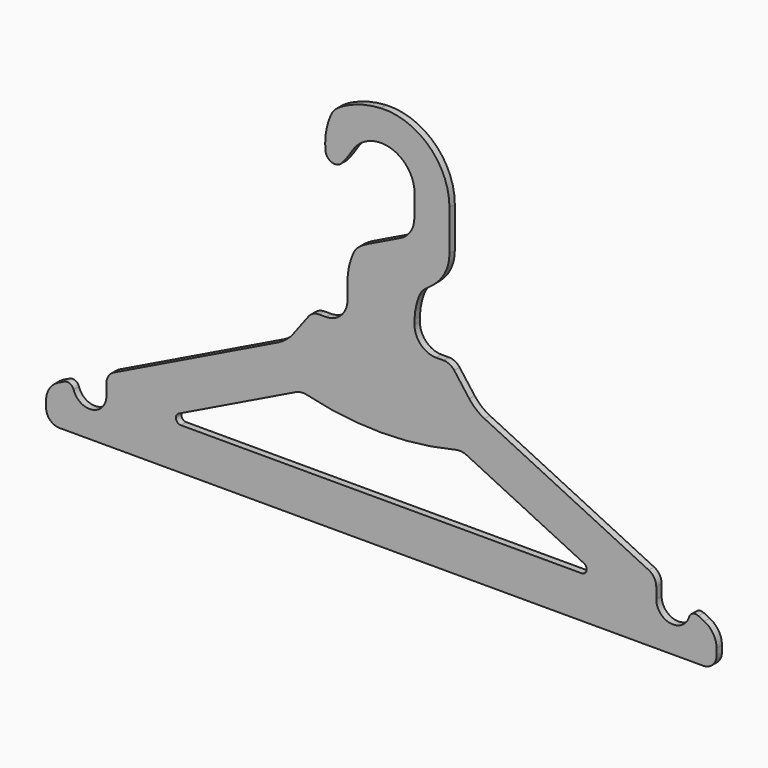
from build123d import *

# Parameters (mm, degrees)
F4_DEPTH = 4
F5_DEPTH = 25
F6_DEPTH = 4


# Not quite as in the source:
# - ends of sketch curves that miss each other by under 0.0002 mm in the source are joined


with BuildPart() as f4:
    # F1 (on Front) → F4 (new body)
    with BuildSketch(Plane.XZ):
        with BuildLine():
            Line((-192, 0), (0, 0))
            Line((0, 0), (192, 0))
            ThreePointArc((192, 0), (197.656854, 2.343146), (200, 8))
            Line((200, 8), (200, 11.867938))
            ThreePointArc((200, 11.867938), (198.021286, 18.762229), (192.6875, 23.557777))
            Line((192.6875, 23.557777), (189.154629, 25.276638))
            ThreePointArc((189.154629, 25.276638), (185.814495, 25.350114), (183.583668, 22.863087))
            ThreePointArc((183.583668, 22.863087), (172.535276, 15.933925), (164.031264, 25.821393))
            Line((164.031264, 25.821393), (164.031264, 32.495654))
            ThreePointArc((164.031264, 32.495654), (162.813594, 36.738295), (159.531264, 39.689401))
            Line((159.531264, 39.689401), (61.560664, 87.355393))
            ThreePointArc((61.560664, 87.355393), (56.583657, 90.555592), (52.498164, 94.835853))
            Line((52.498164, 94.835853), (43.525054, 106.8))
            ThreePointArc((43.525054, 106.8), (40.702763, 109.155418), (37.125054, 110))
            Line((37.125054, 110), (0, 110))
            Line((0, 110), (-37.125054, 110))
            ThreePointArc((-37.125054, 110), (-40.702763, 109.155418), (-43.525054, 106.8))
            Line((-43.525054, 106.8), (-52.498164, 94.835853))
            ThreePointArc((-52.498164, 94.835853), (-56.583657, 90.555592), (-61.560664, 87.355393))
            Line((-61.560664, 87.355393), (-159.531264, 39.689401))
            ThreePointArc((-159.531264, 39.689401), (-162.813594, 36.738295), (-164.031264, 32.495654))
            Line((-164.031264, 32.495654), (-164.031264, 25.821393))
            ThreePointArc((-164.031264, 25.821393), (-172.535276, 15.933925), (-183.583668, 22.863087))
            ThreePointArc((-183.583668, 22.863087), (-185.814495, 25.350114), (-189.154629, 25.276638))
            Line((-189.154629, 25.276638), (-192.6875, 23.557777))
            ThreePointArc((-192.6875, 23.557777), (-198.021286, 18.762229), (-200, 11.867938))
            Line((-200, 11.867938), (-200, 8))
            ThreePointArc((-200, 8), (-197.656854, 2.343146), (-192, 0))
        make_face()
    extrude(amount=F4_DEPTH)

    # F2 (on Front) → F5 (cut)
    with BuildSketch(Plane.XZ):
        with BuildLine():
            Line((-51.048831, 64.667832), (-120.869649, 30.697655))
            ThreePointArc((-120.869649, 30.697655), (-122.480586, 27.326563), (-119.557149, 25))
            Line((-119.557149, 25), (0, 25))
            Line((0, 25), (119.557149, 25))
            ThreePointArc((119.557149, 25), (122.480586, 27.326563), (120.869649, 30.697655))
            Line((120.869649, 30.697655), (51.048831, 64.667832))
            ThreePointArc((51.048831, 64.667832), (47.725881, 65.620153), (44.277223, 65.384214))
            ThreePointArc((44.277223, 65.384214), (22.301694, 61.350993), (0, 60))
            ThreePointArc((0, 60), (-22.301694, 61.350993), (-44.277223, 65.384214))
            ThreePointArc((-44.277223, 65.384214), (-47.725881, 65.620153), (-51.048831, 64.667832))
        make_face()
    extrude(amount=F5_DEPTH, mode=Mode.SUBTRACT)

    # F3 (on Front) → F6 (join)
    with BuildSketch(Plane.XZ):
        with BuildLine():
            ThreePointArc((32.807421, 110), (23.615033, 113.807612), (19.807421, 123))
            Line((19.807421, 123), (19.807421, 123.364001))
            ThreePointArc((19.807421, 123.364001), (19.788107, 124.597592), (19.807421, 125.831184))
            ThreePointArc((19.807421, 125.831184), (20.585942, 132.486795), (22.480947, 138.914252))
            ThreePointArc((22.480947, 138.914252), (24.415358, 142.253814), (27.26686, 144.854497))
            ThreePointArc((27.26686, 144.854497), (31.010569, 147.694728), (34.369154, 150.981394))
            ThreePointArc((34.369154, 150.981394), (39.024435, 158.572921), (40.648173, 167.328856))
            Line((40.648173, 167.328856), (40.648173, 191.46438))
            ThreePointArc((40.648173, 191.46438), (28.559651, 219.648447), (-0.192579, 230.31537))
            ThreePointArc((-0.192579, 230.31537), (-10.806995, 228.704114), (-20.884382, 225.001649))
            ThreePointArc((-20.884382, 225.001649), (-23.281785, 223.734658), (-25.589387, 222.310657))
            ThreePointArc((-25.589387, 222.310657), (-28.274964, 219.911622), (-30.175546, 216.85295))
            ThreePointArc((-30.175546, 216.85295), (-33.010101, 207.16869), (-33.29219, 197.082064))
            ThreePointArc((-33.29219, 197.082064), (-29.366219, 192.282166), (-23.415491, 194.026042))
            ThreePointArc((-23.415491, 194.026042), (-20.19782, 198.150829), (-17.303522, 202.508616))
            ThreePointArc((-17.303522, 202.508616), (5.233812, 211.361001), (19.855826, 192.060927))
            Line((19.855826, 192.060927), (19.688097, 178.809665))
            ThreePointArc((19.688097, 178.809665), (17.438365, 171.242723), (11.55125, 165.983274))
            Line((11.55125, 165.983274), (-7.491858, 156.718162))
            ThreePointArc((-7.491858, 156.718162), (-9.889261, 155.45117), (-12.196863, 154.027169))
            ThreePointArc((-12.196863, 154.027169), (-14.846969, 151.670161), (-16.738426, 148.670005))
            ThreePointArc((-16.738426, 148.670005), (-19.319365, 140.78615), (-20.192579, 132.536671))
            Line((-20.192579, 132.536671), (-20.192579, 123))
            ThreePointArc((-20.192579, 123), (-24.000191, 113.807612), (-33.192579, 110))
            Line((-33.192579, 110), (32.807421, 110))
        make_face()
        with BuildLine():
            ThreePointArc((19.807421, 125.831184), (19.788107, 124.597592), (19.807421, 123.364001))
            Line((19.807421, 123.364001), (19.807421, 125.831184))
        make_face()
    extrude(amount=F6_DEPTH)


solid = f4.part
